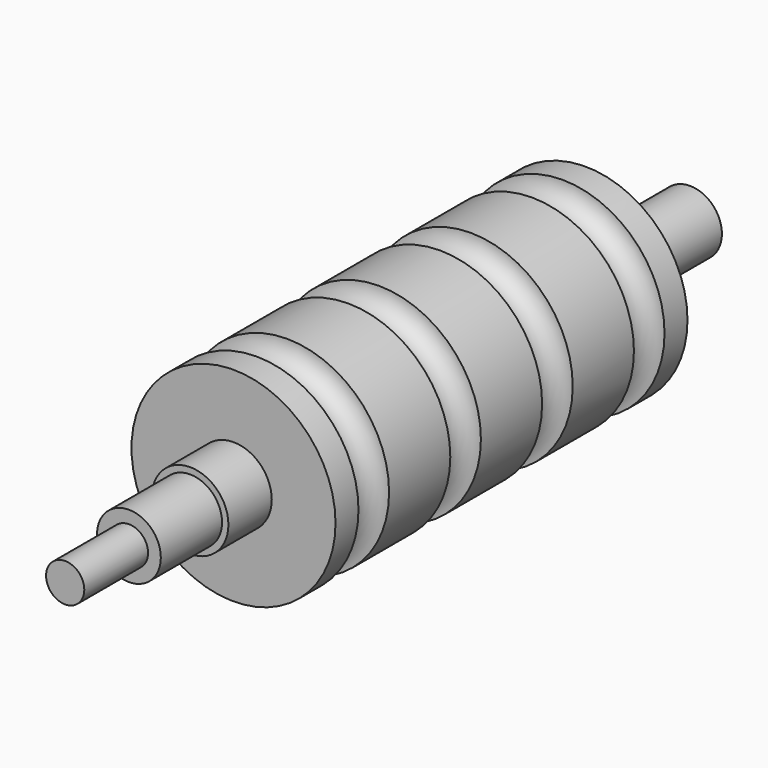
from build123d import *

# Parameters (mm, degrees)
F0_R          = 16
F1_DEPTH      = 34.5
F2_R          = 3
F4_R          = 6
F5_DEPTH      = 43
F5_DEPTH_BACK = 43
F6_R          = 5
F7_DEPTH      = 55
F7_DEPTH_BACK = 55
F8_R          = 3
F9_DEPTH      = 12.5


# Not quite as in the source:
# - a feature names something its author has since deleted; it is built from what else it names


with BuildPart() as f1:
    # F0 (on Front) → F1 (new body, symmetric)
    with BuildSketch(Plane.XZ):
        Circle(F0_R)
    extrude(amount=F1_DEPTH, both=True)

    # F2 (on Right) → F3 (revolve, cut)
    with BuildSketch(Plane.YZ):
        with Locations((-27, 16)):
            Circle(F2_R)
        with Locations((-9, 16)):
            Circle(F2_R)
        with Locations((9, 16)):
            Circle(F2_R)
        with Locations((27, 16)):
            Circle(F2_R)
    revolve(axis=Axis((0, -34.5, 0), (0, -1, 0)), mode=Mode.SUBTRACT)

    # F4 (on Front) → F5 (join, two sides)
    with BuildSketch(Plane.XZ) as f5_sk:
        Circle(F4_R)
    extrude(amount=F5_DEPTH)
    extrude(f5_sk.sketch, amount=-F5_DEPTH_BACK)

    # F6 (on Front) → F7 (join, two sides)
    with BuildSketch(Plane.XZ) as f7_sk:
        Circle(F6_R)
    extrude(amount=F7_DEPTH)
    extrude(f7_sk.sketch, amount=-F7_DEPTH_BACK)

    # F8 (on face) → F9 (join)
    with BuildSketch(Plane.XZ.offset(55)):
        Circle(F8_R)
    extrude(amount=F9_DEPTH)


solid = f1.part
